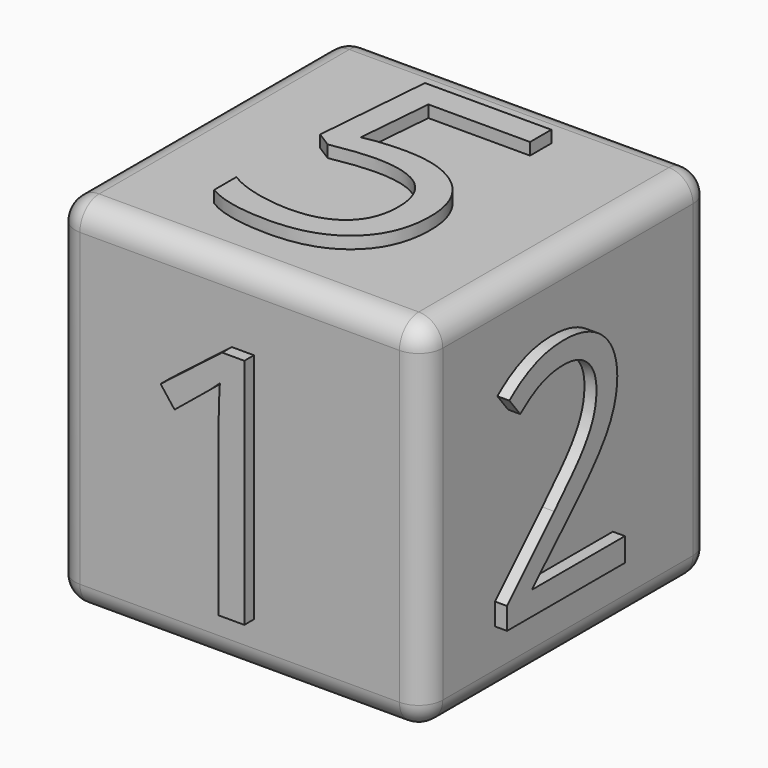
from build123d import *

# Parameters (mm, degrees)
F0_W          = 77.6480846107
F0_H          = 75.5814015865
F1_DEPTH      = 76.2
F2_R          = 5.08
F3_TEXT_SIZE  = 66.2874663249
F4_DEPTH      = 2.54
F5_TEXT_SIZE  = 78.0762794117
F6_DEPTH      = 2.54
F7_TEXT_SIZE  = 72.163490889
F8_DEPTH      = 2.54
F9_TEXT_SIZE  = 68.7755333881
F10_DEPTH     = 2.54
F11_TEXT_SIZE = 75.1807962337
F12_DEPTH     = 2.54


# Not quite as in the source:
# - Text() gives the source's letters only with a copy of the font that has no kerning and outlines rounded to 1/6400 em; it was checked with that copy


with BuildPart() as f1:
    # F0 (on Front) → F1 (new body)
    with BuildSketch(Plane.XZ):
        with Locations((-4.1333567351, -4.4285990298)):
            Rectangle(F0_W, F0_H)
    extrude(amount=F1_DEPTH)

    # F2
    f2_edges = [f1.edges().sort_by_distance(p)[0] for p in [
        (34.690686, -38.1, -42.2193),
        (34.690686, -38.1, 33.362102),
        (34.690686, 0, -4.428599),
        (34.690686, -76.2, -4.428599),
        (-4.133357, -76.2, 33.362102),
        (-42.957399, -76.2, -4.428599),
        (-4.133357, -76.2, -42.2193),
        (-42.957399, -38.1, 33.362102),
        (-4.133357, 0, 33.362102),
        (-42.957399, 0, -4.428599),
        (-4.133357, 0, -42.2193),
        (-42.957399, -38.1, -42.2193),
    ]]
    fillet(f2_edges, radius=F2_R)

    # F3 (on face) → F4 (join)
    with BuildSketch(Plane.YZ.offset(34.6906855702)):
        with Locations((-60.5554655194, -29.067967087)):
            Text('2', F3_TEXT_SIZE, font='Open Sans', text_align=(TextAlign.LEFT, TextAlign.BOTTOM))
    extrude(amount=F4_DEPTH)

    # F5 (on face) → F6 (join)
    with BuildSketch(Plane(origin=(0, 0, 0), x_dir=(-1, 0, 0), z_dir=(0, 1, 0))):
        with Locations((-21.1365576833, -32.1206077933)):
            Text('3', F5_TEXT_SIZE, font='Open Sans', text_align=(TextAlign.LEFT, TextAlign.BOTTOM))
    extrude(amount=F6_DEPTH)

    # F7 (on face) → F8 (join)
    with BuildSketch(Plane(origin=(-42.9573990405, 0, 0), x_dir=(0, -1, 0), z_dir=(-1, 0, 0))):
        with Locations((15.1238432154, -30.2476827055)):
            Text('4', F7_TEXT_SIZE, font='Open Sans', text_align=(TextAlign.LEFT, TextAlign.BOTTOM))
    extrude(amount=F8_DEPTH)

    # F9 (on face) → F10 (join)
    with BuildSketch(Plane.XZ.offset(76.2)):
        with Locations((-25.1250918955, -31.7112803459)):
            Text('1', F9_TEXT_SIZE, font='Open Sans', text_align=(TextAlign.LEFT, TextAlign.BOTTOM))
    extrude(amount=F10_DEPTH)

    # F11 (on face) → F12 (join)
    with BuildSketch(Plane.XY.offset(33.3621017635)):
        with Locations((-25.8036199957, -64.1107112169)):
            Text('5', F11_TEXT_SIZE, font='Open Sans', text_align=(TextAlign.LEFT, TextAlign.BOTTOM))
    extrude(amount=F12_DEPTH)


solid = f1.part
